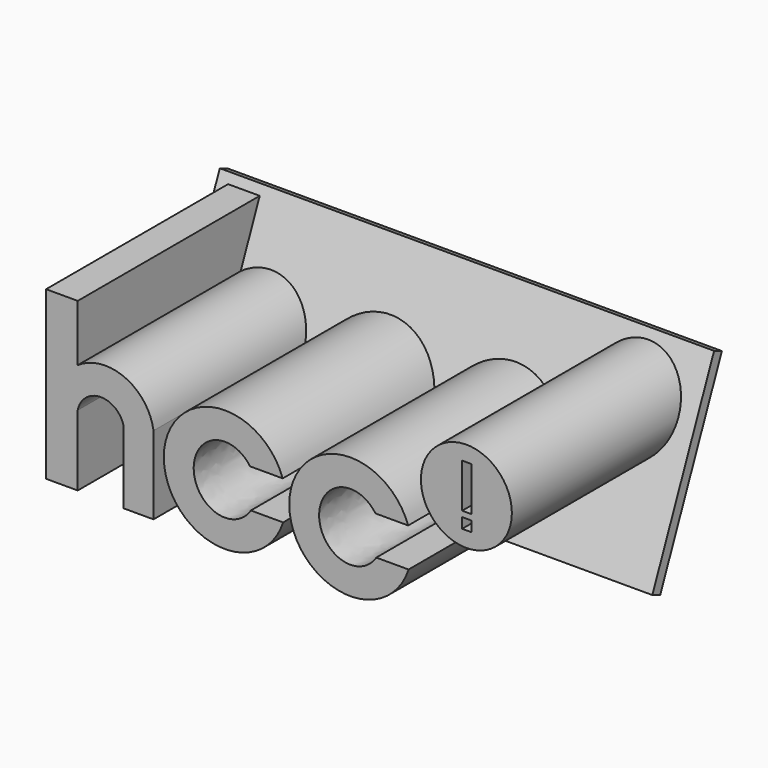
from build123d import *

# Parameters (mm, degrees)
F1_DEPTH = 40
F0_R     = 6.439210956
F0_W     = 1.3290867209
F0_H     = 1.4619943686
F0_H_2   = 6.2467027456
F4_DEPTH = 35
F5_DEPTH = 37.5


# Not quite as in the source:
# - a feature of the source that left no trace in its solid (it failed there, or was rolled back) is left out


with BuildPart() as f1:
    # F0 (on Front) → F1 (new body)
    with BuildSketch(Plane.XZ):
        with BuildLine():
            Line((-28.9235636592, -22.6464916631), (-28.9235636592, -14.6353691816))
            Line((-28.9235636592, -14.6353691816), (-33.4055324317, -14.6353691816))
            Line((-33.4055324317, -14.6353691816), (-33.4055324317, -38.274616003))
            Line((-33.4055324317, -38.274616003), (-28.9235636592, -38.274616003))
            Line((-28.9235636592, -38.274616003), (-28.9235636592, -28.2712467597))
            ThreePointArc((-28.9235636592, -28.2712467597), (-25.7717760928, -25.5693559916), (-22.441348061, -28.0477078049))
            Line((-22.441348061, -28.0477078049), (-22.441348061, -38.3863858879))
            Line((-22.441348061, -38.3863858879), (-18.1943774223, -38.3863858879))
            Line((-18.1943774223, -38.3863858879), (-18.1943774223, -27.3266518489))
            ThreePointArc((-18.1943774223, -27.3266518489), (-22.2574435973, -22.0028437608), (-28.9235636592, -22.6464916631))
        make_face()
    extrude(amount=F1_DEPTH)



with BuildPart() as f1b:
    # F0 (on Front) → F1, piece 2 (new body)
    with BuildSketch(Plane.XZ):
        with BuildLine():
            Line((-4.5282388961, -27.3266518489), (0.1030723041, -27.3266518489))
            ThreePointArc((0.1030723041, -27.3266518489), (-16.733518709, -30.2407605391), (0.1616515454, -32.7934157206))
            Line((0.1616515454, -32.7934157206), (-4.4119914159, -32.7934157206))
            add(Edge.make_bspline(
                [(-4.5282388961, -27.3266518489), (-12.8162053862, -15.3670668623), (-12.4996053357, -30.255800054), (-12.1830052852, -45.1445332456), (-4.4119914159, -32.7934157206)],
                knots=[5.3507793797, 5.3507793797, 5.3507793797, 7.8767470991, 7.8767470991, 10.4027148184, 10.4027148184, 10.4027148184], degree=2, weights=[1, 0.3029746472, 1, 0.3029746472, 1]))
        make_face()
    extrude(amount=F1_DEPTH)


with BuildPart() as f1c:
    # F0 (on Front) → F1, piece 3 (new body)
    with BuildSketch(Plane.XZ):
        with BuildLine():
            Line((13.2356253529, -27.420745464), (17.8669365531, -27.420745464))
            ThreePointArc((17.8669365531, -27.420745464), (1.03034554, -30.3348541543), (17.9255157944, -32.8875093358))
            Line((17.9255157944, -32.8875093358), (13.3518728331, -32.8875093358))
            add(Edge.make_bspline(
                [(13.2356253529, -27.420745464), (4.9476588628, -15.4611604775), (5.2642589133, -30.3498936691), (5.5808589638, -45.2386268608), (13.3518728331, -32.8875093358)],
                knots=[5.3507793797, 5.3507793797, 5.3507793797, 7.8767470991, 7.8767470991, 10.4027148184, 10.4027148184, 10.4027148184], degree=2, weights=[1, 0.3029746472, 1, 0.3029746472, 1]))
        make_face()
    extrude(amount=F1_DEPTH)


with BuildPart() as f1d:
    # F0 (on Front) → F1, piece 4 (new body)
    with BuildSketch(Plane.XZ):
        with Locations((26.1134244502, -21.0938840173)):
            Circle(F0_R)
        with Locations((26.1798799038, -24.615961127)):
            Rectangle(F0_W, F0_H, mode=Mode.SUBTRACT)
        with Locations((26.1798799038, -19.964161329)):
            Rectangle(F0_W, F0_H_2, mode=Mode.SUBTRACT)
    extrude(amount=F1_DEPTH)


with BuildPart() as f1_1:
    add(f1.part)

    add(f1b.part)  # F4 merges F1b

    add(f1c.part)  # F4 merges F1c

    add(f1d.part)  # F4 merges F1d
    # F3 (on Right) → F4 (join, symmetric)
    with BuildSketch(Plane.YZ):
        Polygon((-16.8098711706, -39.9690200104), (-5.8749858439, -13.9690200104), (-7.2576762177, -13.3874984458), (-18.1925615444, -39.3874984458), align=None)
    extrude(amount=F4_DEPTH, both=True)

    # F3 (on Right) → F5 (cut, symmetric)
    with BuildSketch(Plane.YZ):
        Polygon((0, -42.0594814209), (0, 0), (-5.8749858439, -13.9690200104), (-16.8098711706, -39.9690200104), (-17.6890617784, -42.0594814209), align=None)
    extrude(amount=F5_DEPTH, both=True, mode=Mode.SUBTRACT)


solid = f1_1.part
